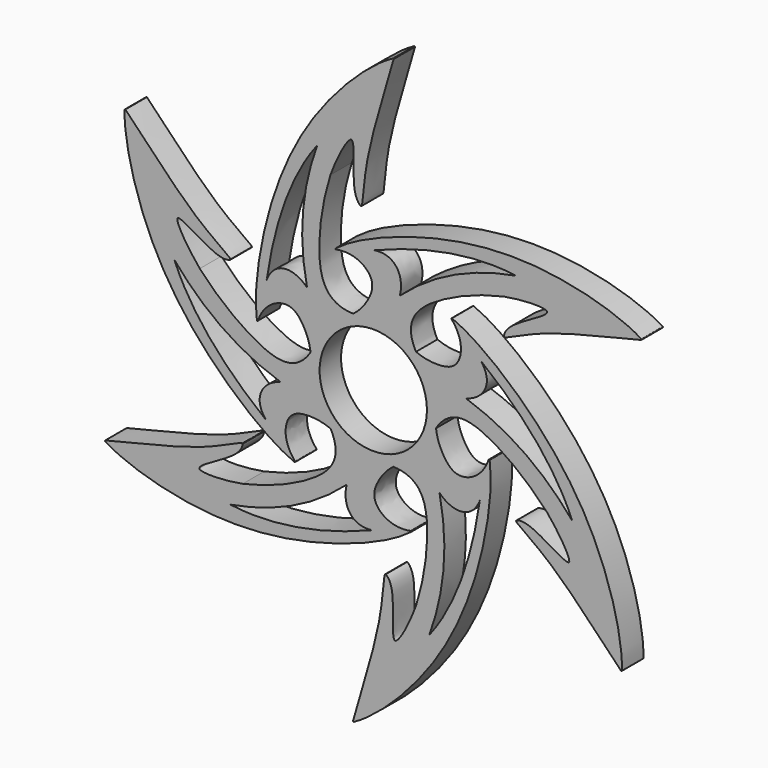
from build123d import *

# Parameters (mm, degrees)
F1_DEPTH = 5
F2_R     = 0.1
F4_DEPTH = 5.0010001
F5_COUNT = 6
F6_R     = 10
F7_DEPTH = 5.0010001


with BuildPart() as f1:
    # F0 (on Front) → F1 (new body)
    with BuildSketch(Plane.XZ):
        with BuildLine():
            add(Edge.make_bspline(
                [(51.4299380785, 69.6398660905), (53.0321225524, 70.7320943475), (54.7707125926, 72.7136397651), (56.7973254875, 77.4860742916), (52.0885102869, 80.4426129453), (48.5283583403, 79.5498266816)],
                knots=[0, 0, 0, 0, 0.3156117959, 0.6039196508, 1, 1, 1, 1], degree=3))
            ThreePointArc((51.4299380785, 69.6398660905), (53.4137257355, 47.3808668637), (64.3568262458, 66.8653994799))
            add(Edge.make_bspline(
                [(80.200470984, 82.0919126272), (75.8858137021, 81.1493070976), (68.6659873555, 78.3723429449), (62.1077178348, 73.2985991021), (62.9236698151, 68.9483731985), (64.3568262458, 66.8653994799)],
                knots=[0, 0, 0, 0, 0.4073616071, 0.7167578132, 1, 1, 1, 1], degree=3))
            add(Edge.make_bspline(
                [(80.200470984, 75.4947587848), (80.317677755, 77.4532729071), (85.7258629469, 80.0656308743), (88.7004136873, 82.0912316882), (87.4140077522, 82.7830822096), (83.6354113268, 82.7003273719), (80.200470984, 82.0919126272)],
                knots=[0, 0, 0, 0, 0.3397411513, 0.5579382535, 0.656937119, 1, 1, 1, 1], degree=3))
            add(Edge.make_bspline(
                [(80.200470984, 75.4947587848), (80.7091168559, 75.2306922033), (87.2229583878, 79.4110527988), (103.8703322411, 82.6360732317), (106.0113359135, 83.3618352191)],
                knots=[0, 0, 0, 0, 0.383355774, 1, 1, 1, 1], degree=3))
            add(Edge.make_bspline(
                [(48.5283583403, 79.5498266816), (51.5742988052, 82.0489429229), (63.5862721662, 87.4108306334), (85.1171760365, 90.7887603888), (101.6252242315, 86.1295230148), (106.0113359135, 83.3618352191)],
                knots=[0, 0, 0, 0, 0.2979661896, 0.6577535061, 1, 1, 1, 1], degree=3))
        make_face()
    extrude(amount=F1_DEPTH)

    # F2
    f2_edges = [f1.edges().sort_by_distance(p)[0] for p in [
        (106.011336, -2.5, 83.361835),
        (80.200471, -2.5, 75.494759),
        (48.528358, -2.5, 79.549827),
    ]]
    fillet(f2_edges, radius=F2_R)

    # F3 (on face) → F4 (cut, through all)
    with BuildSketch(Plane.XZ.offset(5)):
        with BuildLine():
            add(Edge.make_bspline(
                [(56.0287125409, 81.8370580673), (64.8499652743, 85.3655561805), (74.1217285395, 87.402202189), (82.4915021658, 86.2456858158)],
                knots=[0, 0, 0, 0, 26.8275088921, 26.8275088921, 26.8275088921, 26.8275088921], degree=3))
            add(Edge.make_bspline(
                [(56.0287125409, 81.8370580673), (60.0690767169, 82.4542790651), (61.6743154824, 79.1906788945), (60.8096048236, 75.9270787239)],
                knots=[0, 0, 0, 0, 7.6016305395, 7.6016305395, 7.6016305395, 7.6016305395], degree=3))
            add(Edge.make_bspline(
                [(60.8096048236, 75.9270787239), (67.337334156, 81.749111414), (74.5523646474, 84.8342850804), (82.4915021658, 86.2456858158)],
                knots=[0, 0, 0, 0, 24.012045408, 24.012045408, 24.012045408, 24.012045408], degree=3))
        make_face()
    extrude(amount=-F4_DEPTH, mode=Mode.SUBTRACT)

    # F5: F1 ×6 about axis
    f5_axis = Axis((55.8683490202, 0, 58.8175302467), (0, 1, 0))


with BuildPart() as f1_1:
    add(f1.part)
    for i in range(1, F5_COUNT):
        add(f1.part.rotate(f5_axis, i * 360 / F5_COUNT))

    # F6 (on face) → F7 (cut, through all)
    with BuildSketch(Plane.XZ.offset(5)):
        with Locations((55.8683490202, 58.8175302467)):
            Circle(F6_R)
    extrude(amount=-F7_DEPTH, mode=Mode.SUBTRACT)


solid = f1_1.part
